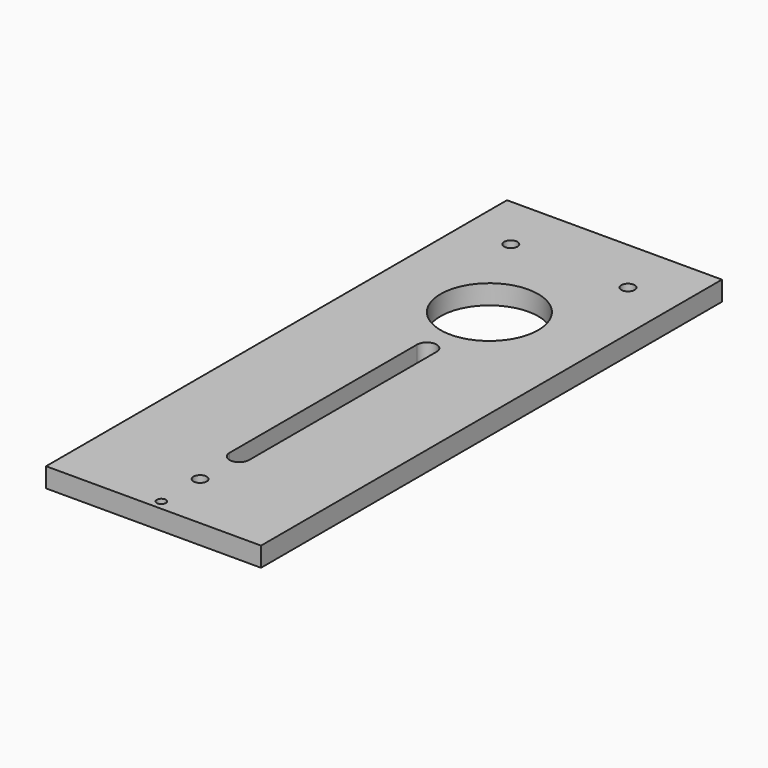
from build123d import *

# Parameters (mm, degrees)
F1_W     = 69.85
F1_H     = 187.2107
F1_R     = 1.4732
F1_R_2   = 2.15265
F1_R_3   = 15.875
F2_DEPTH = 6.35


# Not quite as in the source:
# - a variable given as a bare number and used for a length is read in inches; the dataset says mm whatever the document's units were


with BuildPart() as f2:
    # F1 (on Top) → F2 (new body)
    with BuildSketch(Plane.XY):
        Rectangle(F1_W, F1_H)
        with Locations((0, -90.43035)):
            Circle(F1_R, mode=Mode.SUBTRACT)
        with Locations((0, -74.66965)):
            Circle(F1_R_2, mode=Mode.SUBTRACT)
        with BuildLine():
            ThreePointArc((-3.175, 17.40535), (0, 20.58035), (3.175, 17.40535))
            Line((3.175, 17.40535), (3.175, -58.79465))
            ThreePointArc((3.175, -58.79465), (0, -61.96965), (-3.175, -58.79465))
            Line((-3.175, -58.79465), (-3.175, 17.40535))
        make_face(mode=Mode.SUBTRACT)
        with Locations((-19.05, 75.31735)):
            Circle(F1_R_2, mode=Mode.SUBTRACT)
        with Locations((0, 42.80535)):
            Circle(F1_R_3, mode=Mode.SUBTRACT)
        with Locations((19.05, 75.31735)):
            Circle(F1_R_2, mode=Mode.SUBTRACT)
    extrude(amount=F2_DEPTH)


solid = f2.part
